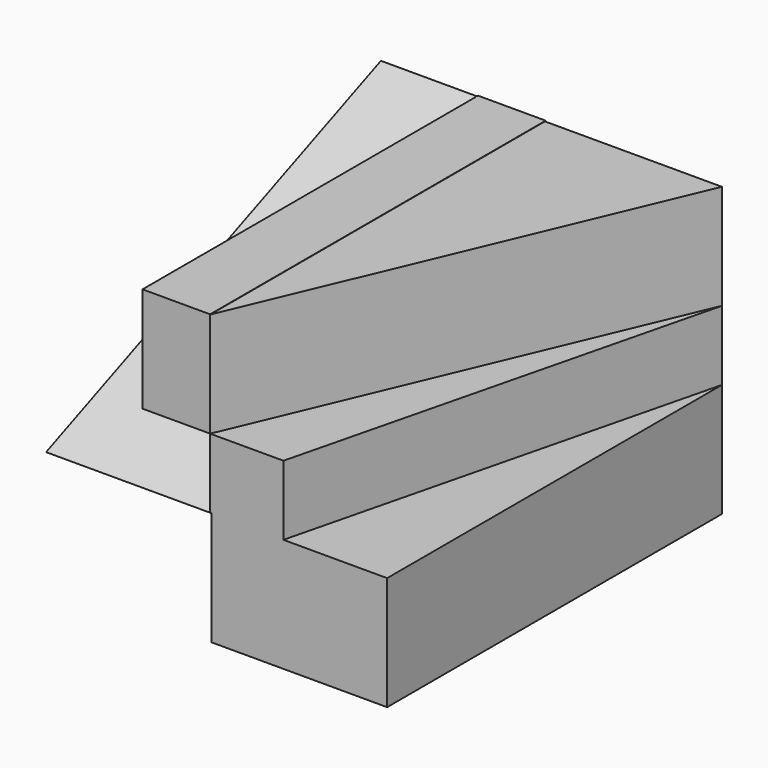
from build123d import *

# Parameters (mm, degrees)
F0_W      = 92.9407775402
F0_H      = 151.2379273772
F1_DEPTH  = 219.7186052799
F3_DEPTH  = 55.0180487335
F4_DEPTH  = 86.1361920834
F6_DEPTH  = 36.5569889545
F8_DEPTH  = 101.3751477003
F9_W      = 86.8442915817
F9_H      = 59.6628896892
F10_DEPTH = 283.972
F12_DEPTH = 86.106
F14_DEPTH = 220.218


with BuildPart() as f1:
    # F0 (on Front) → F1 (new body)
    with BuildSketch(Plane.XZ):
        with Locations((46.4703887701, 75.6189636886)):
            Rectangle(F0_W, F0_H)
    extrude(amount=F1_DEPTH)

    # F2 (on face) → F3 (cut)
    with BuildSketch(Plane.XY.offset(151.2379273772)):
        Polygon((92.9407775402, -219.7186052799), (92.9407775402, 0), (0, -219.7186052799), align=None)
    extrude(amount=-F3_DEPTH, mode=Mode.SUBTRACT)

    # F4 (add): a face of the model
    f4_faces = [f1.faces().sort_by_distance(p)[0] for p in [
        (0, -109.85930264, 75.6189636886),
    ]]
    extrude(f4_faces, amount=F4_DEPTH)

    # F5 (on face) → F6 (cut)
    with BuildSketch(Plane.XY.offset(96.2198786438)):
        Polygon((158.591479063, 33.0015420914), (92.9407775402, 0), (31.3818752766, -248.4212368727), (158.591479063, -248.4212368727), align=None)
        Polygon((158.591479063, 33.0015420914), (92.9407775402, 0), (92.9407775402, -219.7186052799), (38.4944012231, -219.7186052799), (31.3818752766, -248.4212368727), (158.591479063, -248.4212368727), align=None)
    extrude(amount=-F6_DEPTH, mode=Mode.SUBTRACT)

    # F7 (on face) → F8 (cut)
    with BuildSketch(Plane(origin=(-86.1361920834, 0, 0), x_dir=(0, -1, 0), z_dir=(-1, 0, 0))):
        Polygon((29.3830856681, 269.2216336727), (0, 151.2379273772), (219.7186052799, 151.2379273772), (219.7186052799, 65.060840155), (247.8701323271, 54.019369185), (303.3900067808, 195.5738098548), align=None)
    extrude(amount=-F8_DEPTH, mode=Mode.SUBTRACT)

    # F9 (on face) → F10 (cut)
    with BuildSketch(Plane.XZ.offset(219.7186052799)):
        with Locations((-42.7140462925, 29.8314448446)):
            Rectangle(F9_W, F9_H)
    extrude(amount=-F10_DEPTH, mode=Mode.SUBTRACT)

    # F11 (on face) → F12 (cut)
    with BuildSketch(Plane(origin=(-86.1361920834, 0, 0), x_dir=(0, -1, 0), z_dir=(-1, 0, 0))):
        Polygon((219.7186052799, 151.2379273772), (0, 151.2379273772), (219.7186052799, 59.6628896892), align=None)
    extrude(amount=-F12_DEPTH, mode=Mode.SUBTRACT)

    # F13 (on face) → F14 (join)
    with BuildSketch(Plane.XZ.offset(219.7186052799)):
        Polygon((-35.4988574982, 96.2198786438), (-0.0301920834, 96.2198786438), (-0.0301920834, 151.2379273772), (0, 151.2379273772), (0, 151.3858735561), (-35.4988574982, 151.3858735561), align=None)
    extrude(amount=-F14_DEPTH)


solid = f1.part
